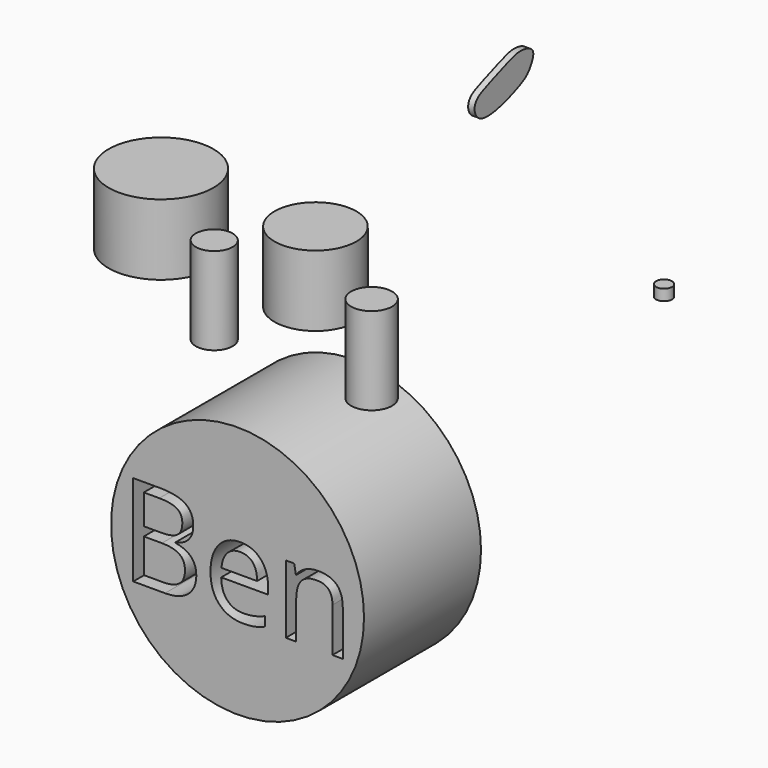
from build123d import *

# Parameters (mm, degrees)
F0_R         = 34.9318151842
F1_DEPTH     = 40.386
F2_R         = 5.090443373
F3_DEPTH     = 24.13
F2_R_2       = 5.6573903538
F4_R         = 14.4784687157
F5_DEPTH     = 19.558
F4_R_2       = 11.2995946928
F6_TEXT_SIZE = 35.1987218236
F7_DEPTH     = 20.32
F9_DEPTH     = 1.778
F10_R        = 2.1821244852
F11_DEPTH    = 3.048


# Not quite as in the source:
# - the program builds the solid bodies; features that only make, move or delete a surface that nothing else refers to are left out
# - Text() gives the source's letters only with a copy of the font that has no kerning and outlines rounded to 1/6400 em; it was checked with that copy


with BuildPart() as f1:
    # F0 (on Front) → F1 (new body)
    with BuildSketch(Plane.XZ):
        with Locations((0, -39.074651897)):
            Circle(F0_R)
    extrude(amount=F1_DEPTH)

    # F6 (on face) → F7 (cut)
    with BuildSketch(Plane.XZ.offset(40.386)):
        with Locations((-32.2593131213, -51.0174170987)):
            Text('Ben', F6_TEXT_SIZE, font='Open Sans', text_align=(TextAlign.LEFT, TextAlign.BOTTOM))
    extrude(amount=-F7_DEPTH, mode=Mode.SUBTRACT)


with BuildPart() as f3:
    # F2 (on Top) → F3 (new body)
    with BuildSketch(Plane.XY):
        with Locations((-24.5612096041, -17.7386514843)):
            Circle(F2_R)
    extrude(amount=F3_DEPTH)


with BuildPart() as f3b:
    # F2 (on Top) → F3, piece 2 (new body)
    with BuildSketch(Plane.XY):
        with Locations((19.1031638533, -17.9867446423)):
            Circle(F2_R_2)
    extrude(amount=F3_DEPTH)


with BuildPart() as f5:
    # F4 (on Top) → F5 (new body)
    with BuildSketch(Plane.XY):
        with Locations((-59.9534027278, 8.1306295469)):
            Circle(F4_R)
    extrude(amount=F5_DEPTH)


with BuildPart() as f5b:
    # F4 (on Top) → F5, piece 2 (new body)
    with BuildSketch(Plane.XY):
        with Locations((-17.028061673, 7.7918502502)):
            Circle(F4_R_2)
    extrude(amount=F5_DEPTH)


with BuildPart() as f9:
    # F8 (on Right) → F9 (new body)
    with BuildSketch(Plane.YZ):
        with BuildLine():
            add(Edge.make_bspline(
                [(54.6823292971, 40.7998003066), (56.641844069, 41.7015645025), (58.2334489508, 42.9489278087), (60.584512732, 47.9319560487), (55.4159464719, 49.4574540332), (51.6437634269, 48.5369796738), (44.4871011129, 45.7217072705), (38.1973092085, 43.382400466), (40.5161150033, 35.5447617349), (51.2902058167, 39.2387528745), (54.6823292971, 40.7998003066)],
                knots=[0, 0, 0, 0, 0.1109098462, 0.2145337712, 0.318453326, 0.423602062, 0.5700958638, 0.695726737, 0.8080035432, 1, 1, 1, 1], degree=3))
        make_face()
    extrude(amount=F9_DEPTH)


with BuildPart() as f11:
    # F10 (on Top) → F11 (new body)
    with BuildSketch(Plane.XY):
        with Locations((38.6803299189, 58.49737674)):
            Circle(F10_R)
    extrude(amount=F11_DEPTH)


solid = Compound([f1.part, f3.part, f3b.part, f5.part, f5b.part, f9.part, f11.part])
